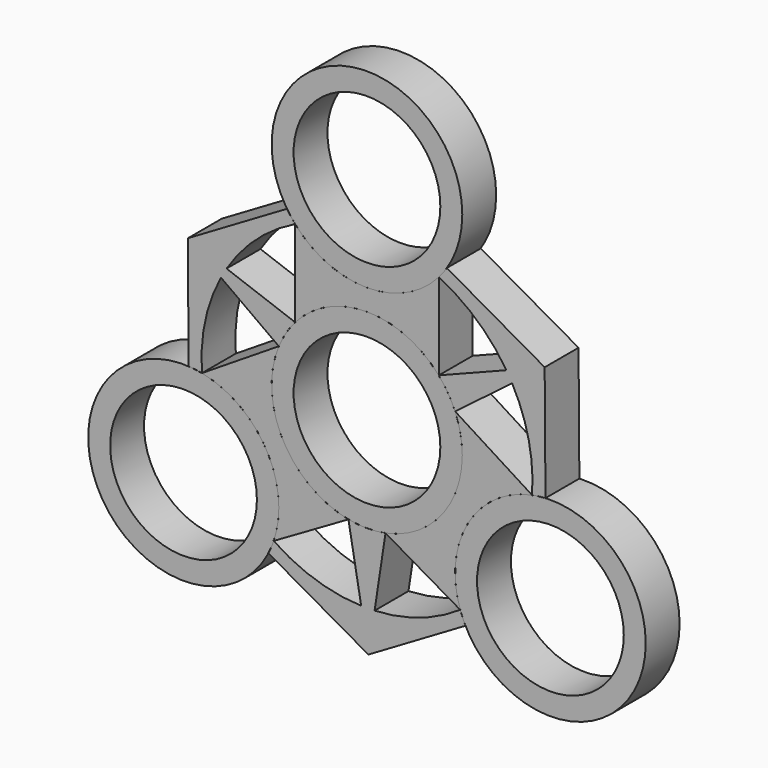
from build123d import *

# Parameters (mm, degrees)
F0_R     = 14.2875
F0_R_2   = 10.9982
F2_DEPTH = 6.35


with BuildPart() as f2:
    # F0 (on Front) → F2 (new body)
    with BuildSketch(Plane.XZ):
        with Locations((27.4963065702, -15.875)):
            Circle(F0_R)
        with Locations((27.4963065702, -15.875)):
            Circle(F0_R_2, mode=Mode.SUBTRACT)
    extrude(amount=F2_DEPTH)


with BuildPart() as f2b:
    # F0 (on Front) → F2, piece 2 (new body)
    with BuildSketch(Plane.XZ):
        Circle(F0_R)
        Circle(F0_R_2, mode=Mode.SUBTRACT)
    extrude(amount=F2_DEPTH)


with BuildPart() as f2c:
    # F0 (on Front) → F2, piece 3 (new body)
    with BuildSketch(Plane.XZ):
        with Locations((0, 31.75)):
            Circle(F0_R)
        with Locations((0, 31.75)):
            Circle(F0_R_2, mode=Mode.SUBTRACT)
    extrude(amount=F2_DEPTH)


with BuildPart() as f2d:
    # F0 (on Front) → F2, piece 4 (new body)
    with BuildSketch(Plane.XZ):
        with Locations((-27.4963065702, -15.875)):
            Circle(F0_R)
        with Locations((-27.4963065702, -15.875)):
            Circle(F0_R_2, mode=Mode.SUBTRACT)
    extrude(amount=F2_DEPTH)


with BuildPart() as f2e:
    # F1 (on Front) → F2, piece 5 (new body)
    with BuildSketch(Plane.XZ):
        with BuildLine():
            Line((24.7404177955, -1.8558083931), (13.2113221809, 5.4400020663))
            ThreePointArc((13.2113221809, 5.4400020663), (14.0158735352, 2.7727144272), (14.2875, 0))
            ThreePointArc((14.2875, 0), (11.0419198775, -9.0668992312), (2.7797258382, -14.0144846682))
            Line((2.7797258382, -14.0144846682), (13.9773861107, -20.4979261146))
            ThreePointArc((13.9773861107, -20.4979261146), (15.1229686136, -8.73125), (24.7404177955, -1.8558083931))
        make_face()
    extrude(amount=F2_DEPTH)


with BuildPart() as f2f:
    # F1 (on Front) → F2, piece 6 (new body)
    with BuildSketch(Plane.XZ):
        with BuildLine():
            ThreePointArc((10.7630316848, 22.3537345077), (0, 17.4625), (-10.7630316848, 22.3537345077))
            Line((-10.7630316848, 22.3537345077), (-10.7630316848, 9.3962654923))
            ThreePointArc((-10.7630316848, 9.3962654923), (0, 14.2875), (10.7630316848, 9.3962654923))
            Line((10.7630316848, 9.3962654923), (10.7630316848, 22.3537345077))
        make_face()
    extrude(amount=F2_DEPTH)


with BuildPart() as f2g:
    # F1 (on Front) → F2, piece 7 (new body)
    with BuildSketch(Plane.XZ):
        with BuildLine():
            ThreePointArc((-2.7797258382, -14.0144846682), (-12.5915712964, -6.751665612), (-13.2113221809, 5.4400020663))
            Line((-13.2113221809, 5.4400020663), (-24.7404177955, -1.8558083931))
            ThreePointArc((-24.7404177955, -1.8558083931), (-16.4621002752, -6.7987150942), (-13.2088065702, -15.875))
            ThreePointArc((-13.2088065702, -15.875), (-13.4022611553, -18.2181901529), (-13.9773861107, -20.4979261146))
            Line((-13.9773861107, -20.4979261146), (-2.7797258382, -14.0144846682))
        make_face()
    extrude(amount=F2_DEPTH)


with BuildPart() as f2h:
    # F1 (on Front) → F2, piece 8 (new body)
    with BuildSketch(Plane.XZ):
        with BuildLine():
            ThreePointArc((2.7797258382, -14.0144846682), (0, -14.2875), (-2.7797258382, -14.0144846682))
            Line((-2.7797258382, -14.0144846682), (-0.8663058881, -24.7947940422))
            ThreePointArc((-0.8663058881, -24.7947940422), (0.1376769661, -24.8095413609), (1.141434315, -24.783652378))
            Line((1.141434315, -24.783652378), (2.7797258382, -14.0144846682))
        make_face()
        with BuildLine():
            ThreePointArc((-13.9773861107, -20.4979261146), (-14.3401220421, -21.4470252075), (-14.7693931554, -22.3679447236))
            Line((-14.7693931554, -22.3679447236), (0.2138989984, -30.880725603))
            Line((0.2138989984, -30.880725603), (14.7592758228, -22.3480753118))
            ThreePointArc((14.7592758228, -22.3480753118), (14.33577822, -21.4367577971), (13.9773861107, -20.4979261146))
            ThreePointArc((13.9773861107, -20.4979261146), (7.8572606656, -23.5328653657), (1.141434315, -24.783652378))
            ThreePointArc((1.141434315, -24.783652378), (0.1376769661, -24.8095413609), (-0.8663058881, -24.7947940422))
            ThreePointArc((-0.8663058881, -24.7947940422), (-7.7265494586, -23.5761050844), (-13.9773861107, -20.4979261146))
        make_face()
    extrude(amount=F2_DEPTH)


with BuildPart() as f2i:
    # F1 (on Front) → F2, piece 9 (new body)
    with BuildSketch(Plane.XZ):
        with BuildLine():
            ThreePointArc((21.7569112787, 11.9234688367), (21.3393208303, 12.6556581808), (20.8970993022, 13.3732396315))
            Line((20.8970993022, 13.3732396315), (10.7630316848, 9.3962654923))
            ThreePointArc((10.7630316848, 9.3962654923), (12.14929693, 7.5184599724), (13.2113221809, 5.4400020663))
            Line((13.2113221809, 5.4400020663), (21.7569112787, 11.9234688367))
        make_face()
        with BuildLine():
            Line((26.6365433603, 15.6256047679), (11.9743630343, 23.9559454599))
            ThreePointArc((11.9743630343, 23.9559454599), (11.3968877171, 23.1335270201), (10.7630316848, 22.3537345077))
            ThreePointArc((10.7630316848, 22.3537345077), (16.454582814, 18.5682255992), (20.8970993022, 13.3732396315))
            ThreePointArc((20.8970993022, 13.3732396315), (21.3393208303, 12.6556581808), (21.7569112787, 11.9234688367))
            ThreePointArc((21.7569112787, 11.9234688367), (24.2480416323, 5.2502166132), (24.7404177955, -1.8558083931))
            ThreePointArc((24.7404177955, -1.8558083931), (25.7437296863, -1.6953973781), (26.7559049388, -1.6066973093))
            Line((26.7559049388, -1.6066973093), (26.6365433603, 15.6256047679))
        make_face()
    extrude(amount=F2_DEPTH)


with BuildPart() as f2j:
    # F1 (on Front) → F2, piece 10 (new body)
    with BuildSketch(Plane.XZ):
        with BuildLine():
            Line((-10.7630316848, 9.3962654923), (-21.0441967437, 13.140551012))
            ThreePointArc((-21.0441967437, 13.140551012), (-21.4779011139, 12.4190201396), (-21.8868764431, 11.6831903628))
            Line((-21.8868764431, 11.6831903628), (-13.2113221809, 5.4400020663))
            ThreePointArc((-13.2113221809, 5.4400020663), (-12.14929693, 7.5184599724), (-10.7630316848, 9.3962654923))
        make_face()
        with BuildLine():
            ThreePointArc((-10.7630316848, 22.3537345077), (-11.4036076442, 23.1424225855), (-11.9865117834, 23.9746420329))
            Line((-11.9865117834, 23.9746420329), (-26.8504423587, 15.255120835))
            Line((-26.8504423587, 15.255120835), (-26.7336388571, -1.6078701482))
            ThreePointArc((-26.7336388571, -1.6078701482), (-25.7326659371, -1.6967692229), (-24.7404177955, -1.8558083931))
            ThreePointArc((-24.7404177955, -1.8558083931), (-24.2765785034, 5.1166428112), (-21.8868764431, 11.6831903628))
            ThreePointArc((-21.8868764431, 11.6831903628), (-21.4779011139, 12.4190201396), (-21.0441967437, 13.140551012))
            ThreePointArc((-21.0441967437, 13.140551012), (-16.5573437666, 18.476651885), (-10.7630316848, 22.3537345077))
        make_face()
    extrude(amount=F2_DEPTH)


solid = Compound([f2.part, f2b.part, f2c.part, f2d.part, f2e.part, f2f.part, f2g.part, f2h.part, f2i.part, f2j.part])
